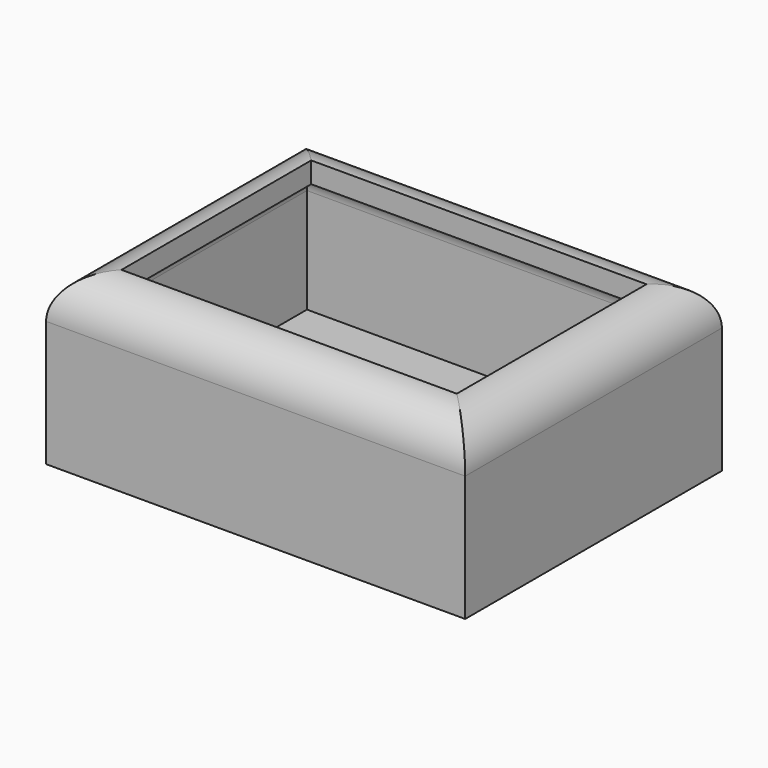
from build123d import *

# Parameters (mm, degrees)
F0_W     = 100
F0_H     = 76.5617211511
F1_DEPTH = 40
F2_R     = 10
F3_T     = -5


# Not quite as in the source:
# - a shell that OpenCascade refuses in one call is made with other operations: the cavity is built on its own and cut out


with BuildPart() as f1:
    # F0 (on Top) → F1 (new body)
    with BuildSketch(Plane.XY):
        with Locations((-141.0329335379, -38.2808605756)):
            Rectangle(F0_W, F0_H)
    extrude(amount=F1_DEPTH)

    # F2
    f2_edges = [f1.edges().sort_by_distance(p)[0] for p in [
        (-141.032934, -76.561721, 40),
        (-91.032934, -38.280861, 40),
        (-141.032934, 0, 40),
        (-191.032934, -38.280861, 40),
    ]]
    fillet(f2_edges, radius=F2_R)

    # F3: a shell. OpenCascade refuses it in one call, so the cavity is built on its own and cut out:
    # the body offset inwards by the wall thickness, plus a prism from it out through each open face.
    f3_core = offset(f1.part, amount=F3_T, mode=Mode.PRIVATE)
    f3_exits = [f3_core.faces().sort_by_distance(p)[0] for p in [
        (-141.032934, -38.280861, 35),
    ]]
    add(f3_core, mode=Mode.SUBTRACT)
    extrude(f3_exits, amount=-F3_T, mode=Mode.SUBTRACT)


solid = f1.part
